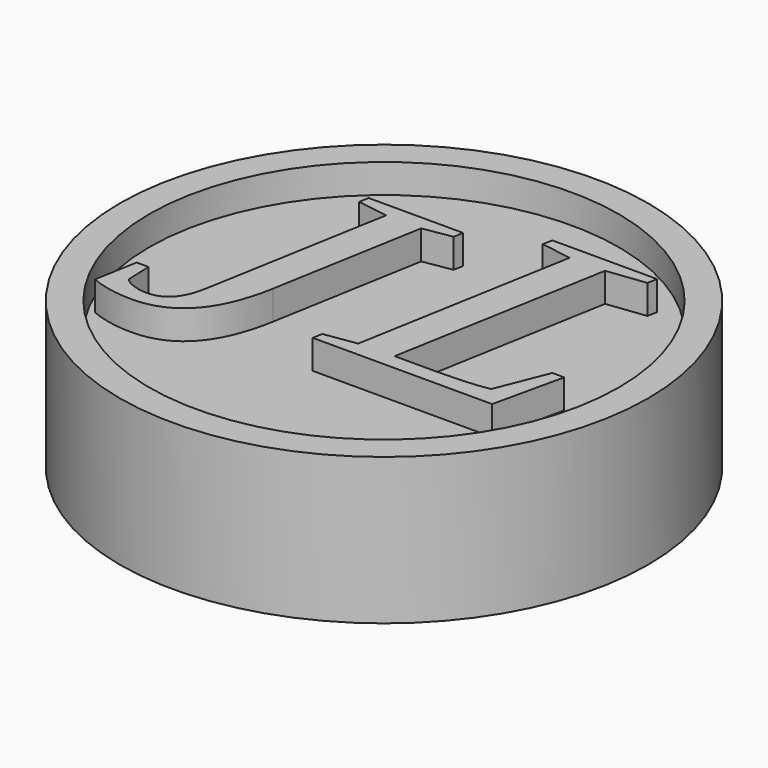
from build123d import *

# Parameters (mm, degrees)
F0_R           = 14.2875
F1_DEPTH       = 6.35
F2_R           = 14.2875
F2_R_2         = 12.7
F3_DEPTH       = 1.5748
F4_TEXT_SIZE   = 20.29166337
F5_DEPTH       = 1.5748
F4_TEXT_SIZE_2 = 20.2847222222
F6_DEPTH       = 1.5748


# Not quite as in the source:
# - Text() gives the source's letters only with a copy of the font that has no kerning and outlines rounded to 1/6400 em; it was checked with that copy


with BuildPart() as f1:
    # F0 (on Top) → F1 (new body)
    with BuildSketch(Plane.XY):
        Circle(F0_R)
    extrude(amount=F1_DEPTH)

    # F2 (on face) → F3 (join)
    with BuildSketch(Plane.XY.offset(6.35)):
        Circle(F2_R)
        Circle(F2_R_2, mode=Mode.SUBTRACT)
    extrude(amount=F3_DEPTH)

    # F4 (on face) → F5 (join)
    with BuildSketch(Plane.XY.offset(6.35)):
        with Locations((-11.0684682539, -6.35)):
            Text('J', F4_TEXT_SIZE, font='Tinos', font_style=FontStyle.ITALIC, text_align=(TextAlign.LEFT, TextAlign.BOTTOM))
    extrude(amount=F5_DEPTH)

    # F4 (on face) → F6 (join)
    with BuildSketch(Plane.XY.offset(6.35)):
        with Locations((0, -4.5258495978)):
            Text('L', F4_TEXT_SIZE_2, font='Tinos', font_style=FontStyle.ITALIC, text_align=(TextAlign.LEFT, TextAlign.BOTTOM))
    extrude(amount=F6_DEPTH)


solid = f1.part
